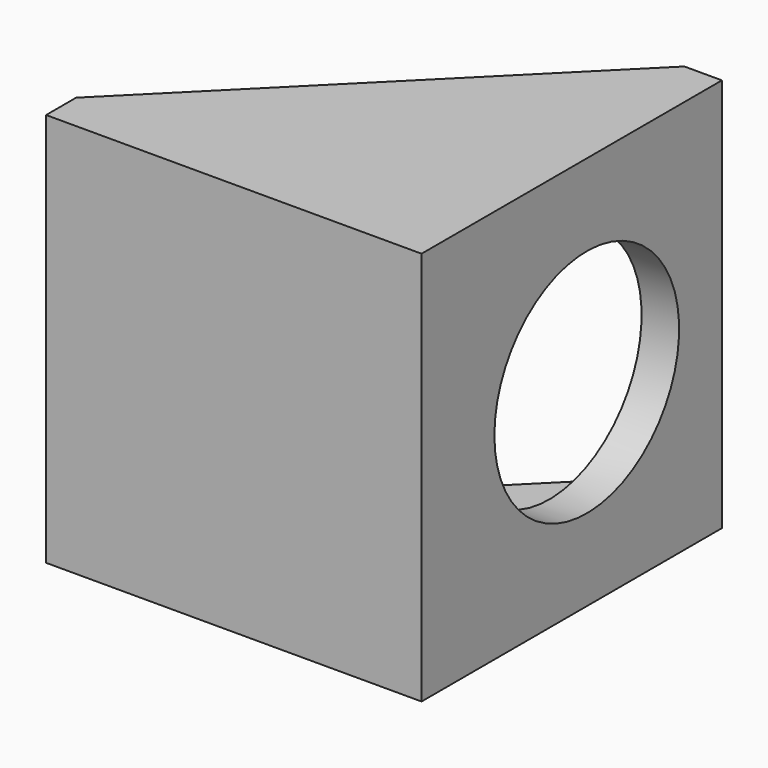
from build123d import *

# Parameters (mm, degrees)
F1_DEPTH = 21
F2_R     = 12.2992849538
F3_DEPTH = 4
F5_DEPTH = 3.6


# Not quite as in the source:
# - a pattern or mirror of a feature is missing from the dataset's text; its kind, count and spacing are read off the source's solid


with BuildPart() as f1:
    # F0 (on Top) → F1 (new body, symmetric)
    with BuildSketch(Plane.XY):
        Polygon((-40, 4), (-40, 0), (0, 0), (0, 40), (-4, 40), (-4, 4), align=None)
    extrude(amount=F1_DEPTH, both=True)

    # F2 (on face) → F3 (cut, through all)
    with BuildSketch(Plane(origin=(-4, 0, 0), x_dir=(0, -1, 0), z_dir=(-1, 0, 0))):
        with Locations((-22, 0)):
            Circle(F2_R)
    extrude(amount=-F3_DEPTH, mode=Mode.SUBTRACT)

    # F4 (on face) → F5 (join)
    with BuildSketch(Plane.XY.offset(21)):
        Polygon((-4, 40), (-40, 4), (-4, 4), align=None)
    f5 = extrude(amount=-F5_DEPTH)

    # F5_copies: F5 across plane
    add(f5.mirror(Plane(origin=(0, 0, 0), x_dir=(-1, 0, 0), z_dir=(0, 0, -1))))


solid = f1.part
